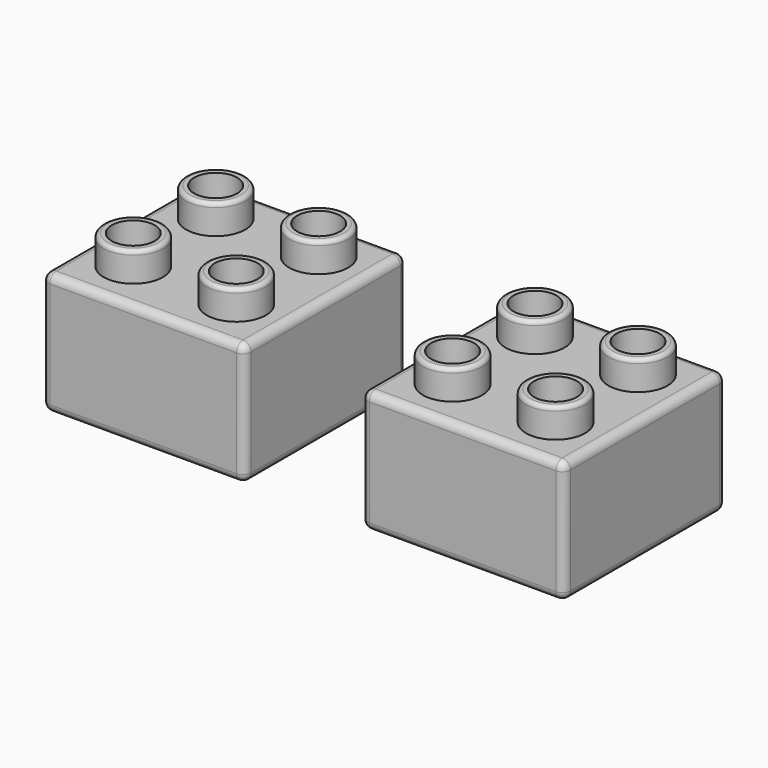
from build123d import *

# Parameters (mm, degrees)
F0_W          = 31.75
F0_H          = 31.75
F5_DEPTH      = 19.177
F1_W          = 28.575
F1_H          = 28.575
F6_DEPTH      = 18.161
F6_DEPTH_BACK = 0.381
F2_R          = 6.5405
F7_DEPTH      = 15.875
F3_R          = 5.461
F8_DEPTH      = 15.875
F8_DEPTH_BACK = 0.635
F4_W          = 1.016
F4_H          = 1.905
F10_DEPTH     = 17.526
F15_ANGLE     = 90
F16_R         = 4.6355
F18_DEPTH     = 4.699
F17_R         = 3.3655
F19_DEPTH     = 4.699
F23_R         = 1.26999
F24_R         = 0.635
F24_2_R       = 0.635
F24_3_R       = 0.635
F24_4_R       = 0.635


# Not quite as in the source:
# - a fillet or chamfer is up to 0.001 mm smaller than in the source, because OpenCascade refuses the exact size


with BuildPart() as f5:
    # F0 (on Top) → F5 (new body)
    with BuildSketch(Plane.XY):
        with Locations((0, -0.3175)):
            Rectangle(F0_W, F0_H)
    extrude(amount=F5_DEPTH)

    # F1 (on face) → F6 (cut, two sides)
    with BuildSketch(Plane.XY) as f6_sk:
        Rectangle(F1_W, F1_H)
    extrude(amount=F6_DEPTH, mode=Mode.SUBTRACT)
    extrude(f6_sk.sketch, amount=-F6_DEPTH_BACK, mode=Mode.SUBTRACT)

    # F23 (radius 1.27 in the source; OpenCascade refuses exactly that, so slightly less here)
    f23_edges = [f5.edges().sort_by_distance(p)[0] for p in [
        (0, -16.1925, 19.177),
        (-15.875, -0.3175, 19.177),
        (0, 15.5575, 19.177),
        (15.875, -0.3175, 19.177),
        (-15.875, -16.1925, 9.5885),
        (15.875, -16.1925, 9.5885),
        (-15.875, 15.5575, 9.5885),
        (15.875, 15.5575, 9.5885),
        (15.875, -0.3175, 0),
        (0, -16.1925, 0),
        (-15.875, -0.3175, 0),
        (0, 15.5575, 0),
    ]]
    fillet(f23_edges, radius=F23_R)


with BuildPart() as f7:
    # F2 (on face) → F7 (new body)
    with BuildSketch(Plane.XY):
        Circle(F2_R)
    extrude(amount=F7_DEPTH)

    # F3 (on face) → F8 (cut, two sides)
    with BuildSketch(Plane.XY) as f8_sk:
        Circle(F3_R)
    extrude(amount=F8_DEPTH, mode=Mode.SUBTRACT)
    extrude(f8_sk.sketch, amount=-F8_DEPTH_BACK, mode=Mode.SUBTRACT)


with BuildPart() as f7_1:
    # F9: moved
    add(f7.part.moved(Location((0, 0, 2.286))))


with BuildPart() as f10:
    # F4 (on face) → F10 (new body)
    with BuildSketch(Plane.XY):
        Rectangle(F4_W, F4_H)
    extrude(amount=F10_DEPTH)


with BuildPart() as f10_1:
    # F11: moved
    add(f10.part.moved(Location((8.0645, 13.8557, 0.635))))


with BuildPart() as f12_1:
    # F12: instance of F10
    add(f10_1.part.mirror(Plane.XZ))


with BuildPart() as f13_1:
    # F13: instance of F12_1
    add(f12_1.part.mirror(Plane.YZ))


with BuildPart() as f13_2:
    # F13: instance of F10
    add(f10_1.part.mirror(Plane.YZ))


with BuildPart() as f15_1:
    # F15: copy of F12_1
    add(f12_1.part.rotate(Axis((0, 0, 4.273429513), (0, 0, -1)), F15_ANGLE))


with BuildPart() as f15_2:
    # F15: copy of F13_1
    add(f13_1.part.rotate(Axis((0, 0, 4.273429513), (0, 0, -1)), F15_ANGLE))


with BuildPart() as f15_3:
    # F15: copy of F10
    add(f10_1.part.rotate(Axis((0, 0, 4.273429513), (0, 0, -1)), F15_ANGLE))


with BuildPart() as f15_4:
    # F15: copy of F13_2
    add(f13_2.part.rotate(Axis((0, 0, 4.273429513), (0, 0, -1)), F15_ANGLE))


with BuildPart() as f18:
    # F16 (on Top) → F18 (new body)
    with BuildSketch(Plane.XY):
        Circle(F16_R)
    extrude(amount=F18_DEPTH)

    # F17 (on Top) → F19 (cut)
    with BuildSketch(Plane.XY):
        Circle(F17_R)
    extrude(amount=F19_DEPTH, mode=Mode.SUBTRACT)


with BuildPart() as f18_1:
    # F20: moved
    add(f18.part.moved(Location((8.0645, 8.0645, 19.05))))


with BuildPart() as f21_1:
    # F21: instance of F18
    add(f18_1.part.mirror(Plane.XZ))


with BuildPart() as f22_1:
    # F22: instance of F18
    add(f18_1.part.mirror(Plane.YZ))

    # F24
    f24_edges = [f22_1.edges().sort_by_distance(p)[0] for p in [
        (-3.429, 8.0645, 23.749),
    ]]
    fillet(f24_edges, radius=F24_R)


with BuildPart() as f22_2:
    # F22: instance of F21_1
    add(f21_1.part.mirror(Plane.YZ))

    # F24#4
    f24_4_edges = [f22_2.edges().sort_by_distance(p)[0] for p in [
        (-3.429, -8.0645, 23.749),
    ]]
    fillet(f24_4_edges, radius=F24_4_R)


with BuildPart() as f18_2:
    add(f18_1.part)

    # F24#2
    f24_2_edges = [f18_2.edges().sort_by_distance(p)[0] for p in [
        (3.429, 8.0645, 23.749),
    ]]
    fillet(f24_2_edges, radius=F24_2_R)


with BuildPart() as f21_1_1:
    add(f21_1.part)

    # F24#3
    f24_3_edges = [f21_1_1.edges().sort_by_distance(p)[0] for p in [
        (3.429, -8.0645, 23.749),
    ]]
    fillet(f24_3_edges, radius=F24_3_R)


with BuildPart() as f25_1:
    # F25: copy of F13_1
    add(f13_1.part.moved(Location((50, 0, 0))))


with BuildPart() as f25_2:
    # F25: copy of F13_2
    add(f13_2.part.moved(Location((50, 0, 0))))


with BuildPart() as f25_3:
    # F25: copy of F21_1
    add(f21_1_1.part.moved(Location((50, 0, 0))))


with BuildPart() as f25_4:
    # F25: copy of F12_1
    add(f12_1.part.moved(Location((50, 0, 0))))


with BuildPart() as f25_5:
    # F25: copy of F10
    add(f10_1.part.moved(Location((50, 0, 0))))


with BuildPart() as f25_6:
    # F25: copy of F18
    add(f18_2.part.moved(Location((50, 0, 0))))


with BuildPart() as f25_7:
    # F25: copy of F15_4
    add(f15_4.part.moved(Location((50, 0, 0))))


with BuildPart() as f25_8:
    # F25: copy of F22_1
    add(f22_1.part.moved(Location((50, 0, 0))))


with BuildPart() as f25_9:
    # F25: copy of F15_3
    add(f15_3.part.moved(Location((50, 0, 0))))


with BuildPart() as f25_10:
    # F25: copy of F5
    add(f5.part.moved(Location((50, 0, 0))))


with BuildPart() as f25_11:
    # F25: copy of F22_2
    add(f22_2.part.moved(Location((50, 0, 0))))


with BuildPart() as f25_12:
    # F25: copy of F15_1
    add(f15_1.part.moved(Location((50, 0, 0))))


with BuildPart() as f25_13:
    # F25: copy of F7
    add(f7_1.part.moved(Location((50, 0, 0))))


with BuildPart() as f25_14:
    # F25: copy of F15_2
    add(f15_2.part.moved(Location((50, 0, 0))))


solid = Compound([f5.part, f7_1.part, f10_1.part, f12_1.part, f13_1.part, f13_2.part, f15_1.part, f15_2.part, f15_3.part, f15_4.part, f22_1.part, f22_2.part, f18_2.part, f21_1_1.part, f25_1.part, f25_2.part, f25_3.part, f25_4.part, f25_5.part, f25_6.part, f25_7.part, f25_8.part, f25_9.part, f25_10.part, f25_11.part, f25_12.part, f25_13.part, f25_14.part])
